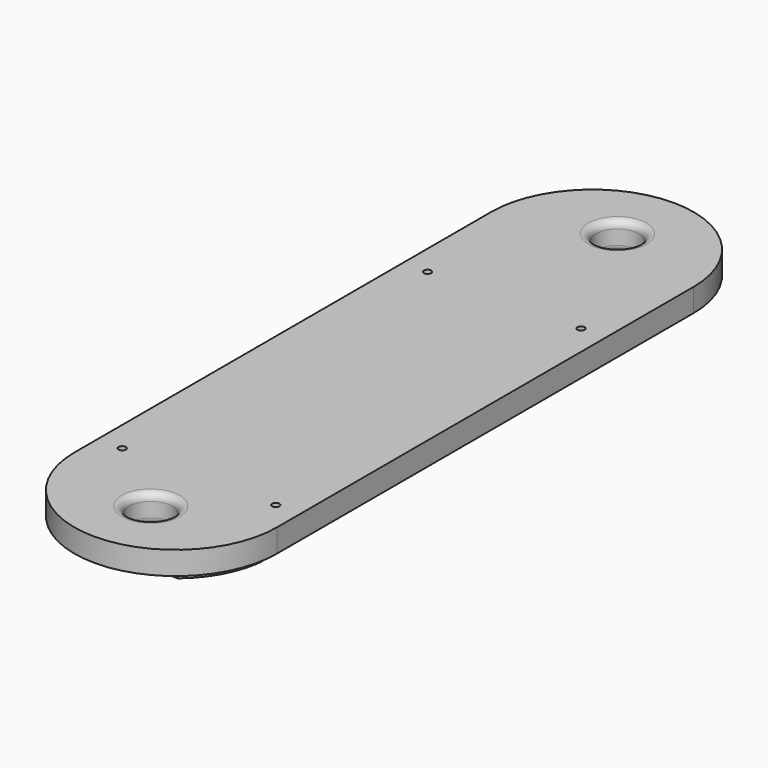
from build123d import *

# Parameters (mm, degrees)
F1_R     = 1.5875
F1_R_2   = 9.525
F2_DEPTH = 12.7
F3_R     = 1.5875
F4_DEPTH = 2.54
F5_R     = 3.175


with BuildPart() as f2:
    # F1 (on Top) → F2 (new body)
    with BuildSketch(Plane.XY):
        with BuildLine():
            ThreePointArc((88.9, 273.05), (44.45, 317.5), (0, 273.05))
            Line((0, 273.05), (0, 44.45))
            ThreePointArc((0, 44.45), (44.45, 0), (88.9, 44.45))
            Line((88.9, 44.45), (88.9, 273.05))
        make_face()
        with Locations((10.853484273, 57.15)):
            Circle(F1_R, mode=Mode.SUBTRACT)
        with Locations((45.2464185655, 29.7988653183)):
            Circle(F1_R_2, mode=Mode.SUBTRACT)
        with Locations((78.2482549548, 57.15)):
            Circle(F1_R, mode=Mode.SUBTRACT)
        with Locations((10.7546523213, 224.79)):
            Circle(F1_R, mode=Mode.SUBTRACT)
        with Locations((43.8685081899, 287.5815033913)):
            Circle(F1_R_2, mode=Mode.SUBTRACT)
        with Locations((78.0730992556, 224.79)):
            Circle(F1_R, mode=Mode.SUBTRACT)
    extrude(amount=-F2_DEPTH)

    # F3 (on face) → F4 (cut)
    with BuildSketch(Plane(origin=(0, 0, -12.7), x_dir=(1, 0, 0), z_dir=(0, 0, -1))):
        with BuildLine():
            Line((0, -44.45), (0, -273.05))
            ThreePointArc((0, -273.05), (44.45, -317.5), (88.9, -273.05))
            Line((88.9, -273.05), (88.9, -44.45))
            ThreePointArc((88.9, -44.45), (44.45, 0), (0, -44.45))
        make_face()
        with Locations((10.7546523213, -224.79)):
            Circle(F3_R, mode=Mode.SUBTRACT)
        with Locations((78.0730992556, -224.79)):
            Circle(F3_R, mode=Mode.SUBTRACT)
        with BuildLine():
            Line((85.725, -241.7593711691), (85.725, -273.05))
            ThreePointArc((85.725, -273.05), (81.8143754619, -290.586506817), (70.8235307648, -304.8))
            Line((70.8235307648, -304.8), (18.0764692352, -304.8))
            ThreePointArc((18.0764692352, -304.8), (7.0856245381, -290.586506817), (3.175, -273.05))
            Line((3.175, -273.05), (3.175, -241.8057641091))
            ThreePointArc((3.175, -241.8057641091), (5.9834868143, -233.8403409002), (13.1668058106, -229.3978761248))
            Line((13.1668058106, -229.3978761248), (15.8026631116, -228.8225635949))
            ThreePointArc((15.8026631116, -228.8225635949), (19.0499999332, -224.7907424019), (15.8041137065, -220.757753291))
            Line((15.8041137065, -220.757753291), (13.1623424416, -220.1801542687))
            ThreePointArc((13.1623424416, -220.1801542687), (5.9820542559, -215.7368852391), (3.175, -207.7732413178))
            Line((3.175, -207.7732413178), (3.175, -73.9505208253))
            ThreePointArc((3.175, -73.9505208253), (6.6440839392, -65.2281250145), (15.1561320755, -61.2708824666))
            ThreePointArc((15.1561320755, -61.2708824666), (19.0324801493, -57.5298939621), (15.9075236341, -53.1417604001))
            Line((15.9075236341, -53.1417604001), (13.1716234423, -52.4694137795))
            ThreePointArc((13.1716234423, -52.4694137795), (5.6434616569, -47.1930989845), (3.648005568, -38.2191994597))
            ThreePointArc((3.648005568, -38.2191994597), (8.5202744008, -24.1354622654), (18.0764692352, -12.7))
            Line((18.0764692352, -12.7), (70.8235307648, -12.7))
            ThreePointArc((70.8235307648, -12.7), (80.4131304814, -24.1946582113), (85.2722946349, -38.3536169954))
            ThreePointArc((85.2722946349, -38.3536169954), (83.1241630177, -47.5004857983), (75.2768639326, -52.6676489864))
            Line((75.2768639326, -52.6676489864), (73.1437855148, -53.1075779034))
            ThreePointArc((73.1437855148, -53.1075779034), (69.850079032, -57.1755421779), (73.1938797929, -61.2024308286))
            Line((73.1938797929, -61.2024308286), (75.4361390988, -61.6360174279))
            ThreePointArc((75.4361390988, -61.6360174279), (82.8206997339, -66.0220738553), (85.725, -74.1050353622))
            Line((85.725, -74.1050353622), (85.725, -207.8391418625))
            ThreePointArc((85.725, -207.8391418625), (82.8133867938, -215.9309577263), (75.4135852009, -220.3124999003))
            Line((75.4135852009, -220.3124999003), (73.2012098097, -220.7361586377))
            ThreePointArc((73.2012098097, -220.7361586377), (69.8500316367, -224.7738395666), (73.1694897792, -228.8376382908))
            Line((73.1694897792, -228.8376382908), (75.5111852948, -229.3050995051))
            ThreePointArc((75.5111852948, -229.3050995051), (82.844993718, -233.7059418761), (85.725, -241.7593711691))
        make_face(mode=Mode.SUBTRACT)
        with Locations((10.853484273, -57.15)):
            Circle(F3_R, mode=Mode.SUBTRACT)
        with Locations((78.2482549548, -57.15)):
            Circle(F3_R, mode=Mode.SUBTRACT)
    extrude(amount=-F4_DEPTH, mode=Mode.SUBTRACT)

    # F5
    f5_edges = [f2.edges().sort_by_distance(p)[0] for p in [
        (35.721419, 29.798865, 0),
        (35.721419, 29.798865, -12.7),
        (34.343508, 287.581503, 0),
        (34.343508, 287.581503, -12.7),
    ]]
    fillet(f5_edges, radius=F5_R)


solid = f2.part
